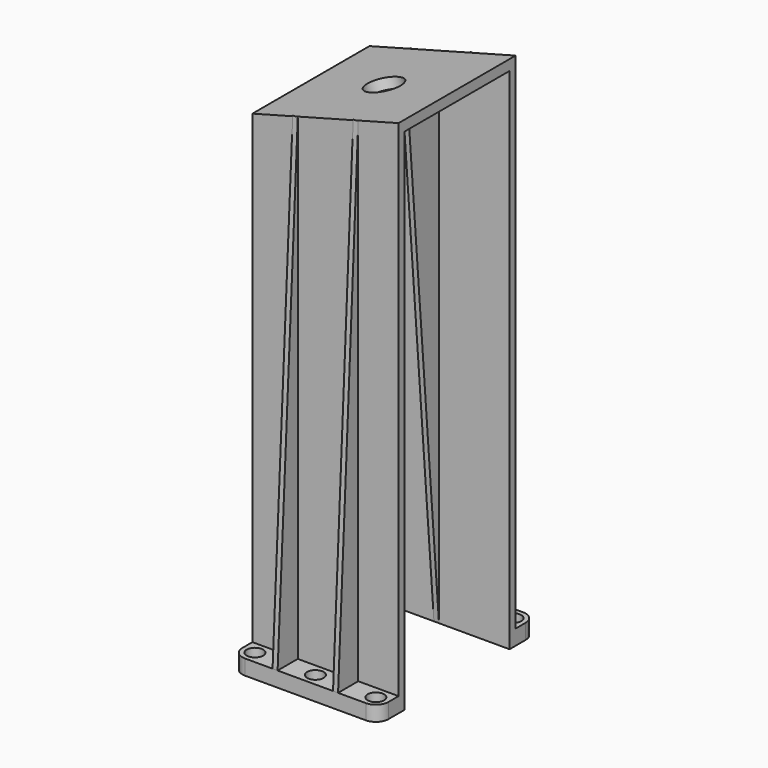
from build123d import *

# Parameters (mm, degrees)
F1_DEPTH  = 29
F0_W      = 28.9777747887
F0_H      = 95.25
F2_DEPTH  = 29
F5_DEPTH  = 3
F6_R      = 2.5
F7_D      = 3.2639
F10_R     = 2.5
F9_W      = 60
F9_H      = 26
F11_DEPTH = 97.505434954
F16_DEPTH = 0.5
F19_DEPTH = 0.5
F22_DEPTH = 0.5
F23_D     = 6.7564


# Not quite as in the source:
# - a feature names something its author has since deleted; it is built from what else it names


with BuildPart() as f1:
    # F0 (on Front) → F1 (new body)
    with BuildSketch(Plane.XZ):
        Polygon((28.9777747887, 7.7645713531), (0, 0), (28.9777747887, 0), align=None)
    extrude(amount=F1_DEPTH)

    # F0 (on Front) → F2 (join)
    with BuildSketch(Plane.XZ):
        Polygon((28.9777747887, 7.7645713531), (0, 0), (28.9777747887, 0), align=None)
        with Locations((14.4888873943, -47.625)):
            Rectangle(F0_W, F0_H)
    extrude(amount=F2_DEPTH)

    # F4 (on face) → F5 (join)
    with BuildSketch(Plane(origin=(0, 0, -95.25), x_dir=(1, 0, 0), z_dir=(0, 0, -1))):
        Polygon((0, 29), (14.4888873943, 29), (28.9777747887, 29), (28.9777747887, 34), (0, 34), align=None)
        Polygon((28.9777747887, 0), (14.4888873943, 0), (0, 0), (0, -5), (28.9777747887, -5), align=None)
    extrude(amount=-F5_DEPTH)

    # F6
    f6_edges = [f1.edges().sort_by_distance(p)[0] for p in [
        (28.977775, -34, -93.75),
        (0, -34, -93.75),
    ]]
    fillet(f6_edges, radius=F6_R)

    # F7 (through all)
    with Locations(Plane(origin=(0, 0, -95.25), x_dir=(1, 0, 0), z_dir=(0, 0, -1))):
        with Locations((2.5, 31.5), (14.4888873943, 31.5), (26.4777747887, 31.5), (2.5, -2.5), (14.4888873943, -2.5), (26.4777747887, -2.5)):
            Hole(F7_D / 2)

    # F10
    f10_edges = [f1.edges().sort_by_distance(p)[0] for p in [
        (28.977775, 5, -93.75),
        (0, 5, -93.75),
    ]]
    fillet(f10_edges, radius=F10_R)

    # F9 (on offset) → F11 (cut, through all)
    with BuildSketch(Plane(origin=(0.5176380902, 0, -1.9318516526), x_dir=(0.9659258263, 0, 0.2588190451), z_dir=(-0.2588190451, 0, 0.9659258263))):
        with Locations((-0.5358983849, -14.5)):
            Rectangle(F9_W, F9_H)
    extrude(amount=-F11_DEPTH, mode=Mode.SUBTRACT)

    # F15 (on plane+point) → F16 (join, symmetric)
    with BuildSketch(Plane.YZ.offset(20.4833310915)):
        Polygon((-29, -92.25), (-29, 5.4884920243), (-34, -92.25), align=None)
        Polygon((5, -92.25), (0, 5.4884920243), (0, -92.25), align=None)
    extrude(amount=F16_DEPTH, both=True)

    # F18 (on plane+point) → F19 (join, symmetric)
    with BuildSketch(Plane.YZ.offset(8.4944436972)):
        Polygon((5, -92.25), (0, 2.2760793288), (0, -92.25), align=None)
        Polygon((-34, -92.25), (-29, -92.25), (-29, 2.2760793288), align=None)
    extrude(amount=F19_DEPTH, both=True)

    # F21 (on plane+point) → F22 (join, symmetric)
    with BuildSketch(Plane.YZ.offset(14.4888873943)):
        Polygon((-27.5, 1.8117333157), (-27.5, -95.25), (-19.5, 1.8117333157), align=None)
        Polygon((-1.5, 1.8117333157), (-9.5, 1.8117333157), (-1.5, -95.25), align=None)
    extrude(amount=F22_DEPTH, both=True)

    # F23 (through all)
    with Locations(Plane(origin=(0, 0, 0), x_dir=(0.9659258263, 0, 0.2588190451), z_dir=(-0.2588190451, 0, 0.9659258263))):
        with Locations((15, -14.5)):
            Hole(F23_D / 2)


solid = f1.part
